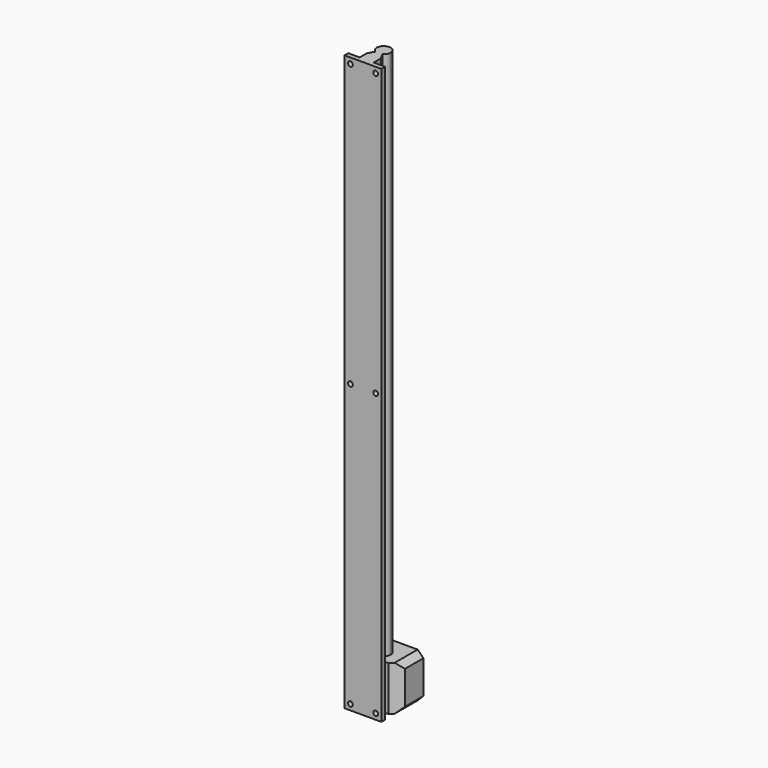
from build123d import *

# Parameters (mm, degrees)
F1_DEPTH = 500
F2_DEPTH = 39
F4_D     = 3.3
F4_DEPTH = 15
F4_TIP   = 0.9914200214
F5_SIZE  = 8
F6_SIZE  = 5
F8_D     = 4.2
F8_DEPTH = 7
F8_TIP   = 1.2618073


with BuildPart() as f1:
    # F0 (on Top) → F1 (new body)
    with BuildSketch(Plane.XY):
        with BuildLine():
            ThreePointArc((3, 17.3038475773), (5.1961524227, 19.5), (6, 22.5))
            ThreePointArc((6, 22.5), (-3, 27.6961524227), (-3, 17.3038475773))
            ThreePointArc((-3, 17.3038475773), (0, 16.5), (3, 17.3038475773))
        make_face()
        with BuildLine():
            ThreePointArc((3, 17.3038475773), (0, 16.5), (-3, 17.3038475773))
            Line((-3, 17.3038475773), (-6.0621778265, 12))
            Line((-6.0621778265, 12), (-6.0621778265, 4))
            Line((-6.0621778265, 4), (6.0621778265, 4))
            Line((6.0621778265, 4), (6.0621778265, 12))
            Line((6.0621778265, 12), (3, 17.3038475773))
        make_face()
        Polygon((6.0621778265, 4), (-6.0621778265, 4), (-16, 4), (-16, 0), (16, 0), (16, 4), align=None)
    extrude(amount=F1_DEPTH)

    # F8
    with Locations(Plane.XZ):
        with Locations((11, 5), (-11, 5), (11, 250), (-11, 250), (11, 495), (-11, 495)):
            Hole(F8_D / 2, depth=F8_DEPTH)
            with Locations((0, 0, -(F8_DEPTH + F8_TIP / 2))):  # 118° drill point
                Cone(0, F8_D / 2, F8_TIP, mode=Mode.SUBTRACT)


with BuildPart() as f2:
    # F0 (on Top) → F2 (new body)
    with BuildSketch(Plane.XY):
        with BuildLine():
            ThreePointArc((-3, 17.3038475773), (-3, 27.6961524227), (6, 22.5))
            ThreePointArc((6, 22.5), (5.1961524227, 19.5), (3, 17.3038475773))
            Line((3, 17.3038475773), (6.0621778265, 12))
            Line((6.0621778265, 12), (20.5, 12))
            Line((20.5, 12), (20.5, 40))
            Line((20.5, 40), (-20.5, 40))
            Line((-20.5, 40), (-20.5, 12))
            Line((-20.5, 12), (-6.0621778265, 12))
            Line((-6.0621778265, 12), (-3, 17.3038475773))
        make_face()
    extrude(amount=F2_DEPTH)

    # F4
    with Locations(Plane(origin=(0, 40, 0), x_dir=(-1, 0, 0), z_dir=(0, 1, 0))):
        with Locations((-12.5, 32), (-12.5, 7), (12.5, 7), (12.5, 32)):
            Hole(F4_D / 2, depth=F4_DEPTH)
            with Locations((0, 0, -(F4_DEPTH + F4_TIP / 2))):  # 118° drill point
                Cone(0, F4_D / 2, F4_TIP, mode=Mode.SUBTRACT)

    # F5
    f5_edges = [f2.edges().sort_by_distance(p)[0] for p in [
        (20.5, 12, 19.5),
        (-20.5, 12, 19.5),
    ]]
    chamfer(f5_edges, length=F5_SIZE)

    # F6
    f6_edges = [f2.edges().sort_by_distance(p)[0] for p in [
        (20.5, 30, 39),
        (20.5, 30, 0),
        (-20.5, 30, 0),
        (-20.5, 30, 39),
    ]]
    chamfer(f6_edges, length=F6_SIZE)


solid = Compound([f1.part, f2.part])
